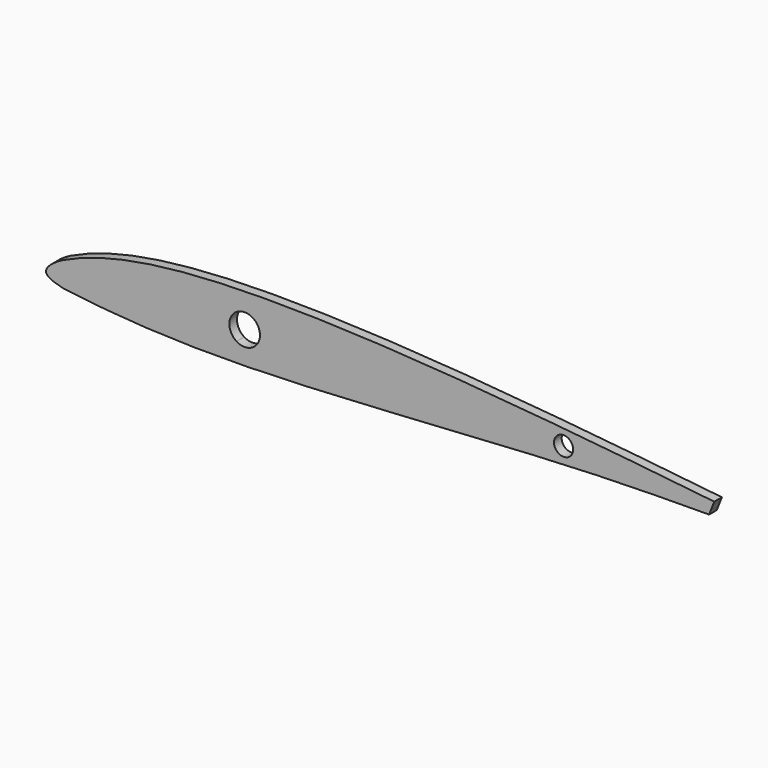
from build123d import *

# Parameters (mm, degrees)
F2_DEPTH = 2.5
F1_R     = 2.5
F3_DEPTH = 3
F4_DEPTH = 3


with BuildPart() as f2:
    # F0 (on Front) → F2 (new body)
    with BuildSketch(Plane.XZ):
        with BuildLine():
            add(Edge.make_bspline(
                [(-96.9805282175, -0.8100506688), (-84.7869920978, 5.1468541776), (-43.2313518226, 10.3846705605), (26.8477938201, 4.0208678603), (73.1462007926, -1.0427900778)],
                knots=[0, 0, 0, 0, 0.374886421, 0.9004696716, 0.9004696716, 0.9004696716, 0.9004696716], degree=3))
            add(Edge.make_bspline(
                [(-97.5447368223, -7.1186651935), (-99.939251346, -6.5508492693), (-102.885147974, -5.168950634), (-100.0067471137, -2.3789404522), (-96.9805282175, -0.8100506688)],
                knots=[0.0564585679, 0.0564585679, 0.0564585679, 0.0564585679, 0.4847104148, 1, 1, 1, 1], degree=3))
            add(Edge.make_bspline(
                [(-96.5428845142, -7.3406707446), (-96.8949965543, -7.2673488468), (-97.22905608, -7.1935231869), (-97.5447368223, -7.1186651935)],
                knots=[0, 0, 0, 0, 0.0564585679, 0.0564585679, 0.0564585679, 0.0564585679], degree=3))
            add(Edge.make_bspline(
                [(-96.5428845142, -7.3406707446), (-80.7020161693, -9.4302402111), (-44.2471235075, -11.1181020976), (27.9226364637, -4.7767282079), (62.4434148738, -4.5021877215), (71.7967184236, -4.4503783305)],
                knots=[0, 0, 0, 0, 0.2987594418, 0.6837410955, 0.8381168975, 0.8381168975, 0.8381168975, 0.8381168975], degree=3))
            Line((71.7967184236, -4.4503783305), (72.2670713195, -3.2626866351))
            add(Edge.make_bspline(
                [(-97.3825784566, -6.0471531808), (-82.3468325761, -8.841713568), (-44.2551066449, -8.6286827794), (32.5707299039, -3.8332069517), (63.1103828262, -3.2710139005), (72.2670713195, -3.2626866351)],
                knots=[0, 0, 0, 0, 0.3131273629, 0.7122131732, 0.9019797674, 0.9019797674, 0.9019797674, 0.9019797674], degree=3))
            add(Edge.make_bspline(
                [(-97.3825784566, -6.0471531808), (-98.6588937786, -5.8946130057), (-100.1661659123, -5.1778479876), (-99.9138553768, -4.2244412327), (-99.8196757147, -4.047003109)],
                knots=[0, 0, 0, 0, 0.4440177242, 0.5425000514, 0.5425000514, 0.5425000514, 0.5425000514], degree=3))
            add(Edge.make_bspline(
                [(-99.8196757147, -4.047003109), (-99.3821638101, -3.2227137691), (-97.9006497107, -2.3042858417), (-96.3385477662, -1.6362179573)],
                knots=[0.5425000514, 0.5425000514, 0.5425000514, 0.5425000514, 1, 1, 1, 1], degree=3))
            add(Edge.make_bspline(
                [(-96.3385477662, -1.6362179573), (-85.7442874691, 3.2900694446), (-41.4192830911, 9.6956733525), (28.5693195485, 2.5855104747), (72.7689680214, -1.9953434339)],
                knots=[0, 0, 0, 0, 0.384923117, 0.9441251659, 0.9441251659, 0.9441251659, 0.9441251659], degree=3))
            Line((72.7689680214, -1.9953434339), (73.1462007926, -1.0427900778))
        make_face()
        with BuildLine():
            add(Edge.make_bspline(
                [(-96.5428845142, -7.3406707446), (-96.8949965543, -7.2673488468), (-97.22905608, -7.1935231869), (-97.5447368223, -7.1186651935)],
                knots=[0, 0, 0, 0, 0.0564585679, 0.0564585679, 0.0564585679, 0.0564585679], degree=3))
            ThreePointArc((-97.5447368223, -7.1186651935), (-97.052492706, -7.2688477084), (-96.5428845142, -7.3406707446))
        make_face()
        with BuildLine():
            Line((72.2670713195, -3.2626866351), (72.7689680214, -1.9953434339))
            add(Edge.make_bspline(
                [(-96.3385477662, -1.6362179573), (-85.7442874691, 3.2900694446), (-41.4192830911, 9.6956733525), (28.5693195485, 2.5855104747), (72.7689680214, -1.9953434339)],
                knots=[0, 0, 0, 0, 0.384923117, 0.9441251659, 0.9441251659, 0.9441251659, 0.9441251659], degree=3))
            add(Edge.make_bspline(
                [(-99.8196757147, -4.047003109), (-99.3821638101, -3.2227137691), (-97.9006497107, -2.3042858417), (-96.3385477662, -1.6362179573)],
                knots=[0.5425000514, 0.5425000514, 0.5425000514, 0.5425000514, 1, 1, 1, 1], degree=3))
            add(Edge.make_bspline(
                [(-97.3825784566, -6.0471531808), (-98.6588937786, -5.8946130057), (-100.1661659123, -5.1778479876), (-99.9138553768, -4.2244412327), (-99.8196757147, -4.047003109)],
                knots=[0, 0, 0, 0, 0.4440177242, 0.5425000514, 0.5425000514, 0.5425000514, 0.5425000514], degree=3))
            add(Edge.make_bspline(
                [(-97.3825784566, -6.0471531808), (-82.3468325761, -8.841713568), (-44.2551066449, -8.6286827794), (32.5707299039, -3.8332069517), (63.1103828262, -3.2710139005), (72.2670713195, -3.2626866351)],
                knots=[0, 0, 0, 0, 0.3131273629, 0.7122131732, 0.9019797674, 0.9019797674, 0.9019797674, 0.9019797674], degree=3))
        make_face()
    extrude(amount=F2_DEPTH)


with BuildPart() as f2b:
    # F1 (on Front) → F2, piece 2 (new body)
    with BuildSketch(Plane.XZ):
        with BuildLine():
            ThreePointArc((-45.542362095, -1.3708024857), (-51.4789804014, 2.1291274472), (-51.6671168627, -4.7598166753))
            Line((-51.6671168627, -4.7598166753), (-47.385046135, -4.7391830831))
            ThreePointArc((-47.385046135, -4.7391830831), (-46.0331411102, -3.2905337378), (-45.542362095, -1.3708024857))
        make_face()
        with BuildLine():
            Line((-47.385046135, -4.7391830831), (-51.6671168627, -4.7598166753))
            ThreePointArc((-51.6671168627, -4.7598166753), (-49.523087913, -5.3707560487), (-47.385046135, -4.7391830831))
        make_face()
    extrude(amount=F2_DEPTH)


with BuildPart() as f2c:
    # F1 (on Front) → F2, piece 3 (new body)
    with BuildSketch(Plane.XZ):
        with Locations((33.7789729238, -1.0305350879)):
            Circle(F1_R)
    extrude(amount=F2_DEPTH)


with BuildPart() as f3_tool:
    # F3 (cut): a face of the model
    f3_faces = [f2b.part.faces().sort_by_distance(p)[0] for p in [
        (-49.542362095, -2.5, -1.3708024857),
    ]]
    extrude(f3_faces, amount=-F3_DEPTH)


with BuildPart() as f2_1:
    add(f2.part)

    # F3: cut by f3_tool
    add(f3_tool.part, mode=Mode.SUBTRACT)


with BuildPart() as f2b_1:
    add(f2b.part)

    # F3: cut by f3_tool
    add(f3_tool.part, mode=Mode.SUBTRACT)


with BuildPart() as f4_tool:
    # F4 (cut): a face of the model
    f4_faces = [f2c.part.faces().sort_by_distance(p)[0] for p in [
        (33.7789729238, -2.5, -1.0305350879),
    ]]
    extrude(f4_faces, amount=-F4_DEPTH)


with BuildPart() as f2_2:
    add(f2_1.part)

    # F4: cut by f4_tool
    add(f4_tool.part, mode=Mode.SUBTRACT)


with BuildPart() as f2c_1:
    add(f2c.part)

    # F4: cut by f4_tool
    add(f4_tool.part, mode=Mode.SUBTRACT)


solid = f2_2.part
